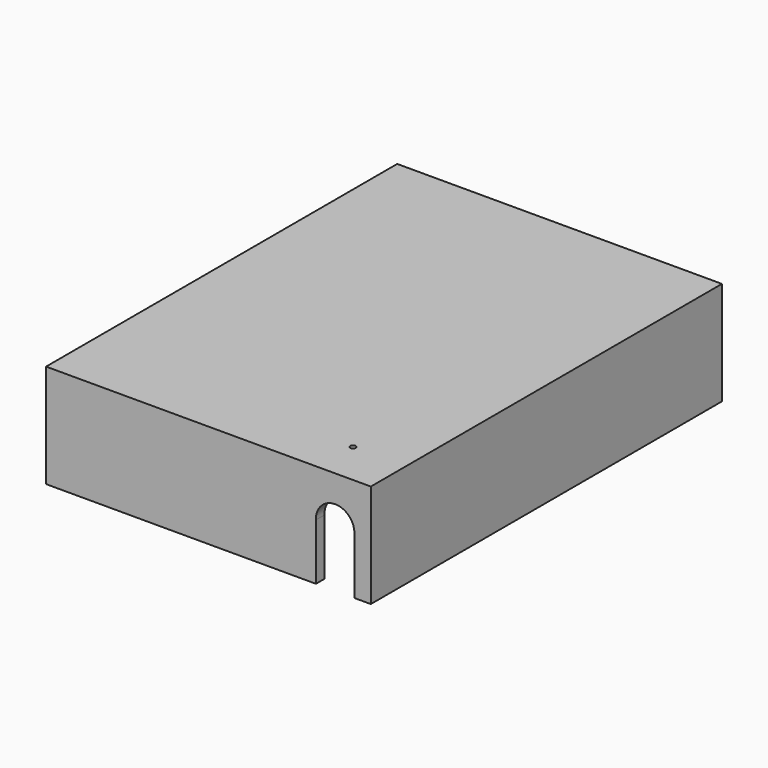
from build123d import *

# Parameters (mm, degrees)
F0_W      = 85
F0_H      = 117
F1_DEPTH  = 4
F2_W      = 2
F2_H      = 5
F3_DEPTH  = 7
F4_W      = 2
F4_H      = 4.0044696238
F5_DEPTH  = 5
F6_R      = 1
F7_R      = 1
F8_R      = 2
F11_W     = 117
F11_H     = 4
F12_DEPTH = 3
F10_W     = 117
F10_H     = 4
F14_DEPTH = 3
F13_W     = 85
F13_H     = 3
F13_W_2   = 3
F13_H_2   = 117
F15_DEPTH = 25
F16_DEPTH = 3
F18_DEPTH = 3
F19_R     = 0.75
F20_DEPTH = 4
F21_DEPTH = 3
F23_DEPTH = 3


# Not quite as in the source:
# - a feature names something its author has since deleted; it is built from what else it names


with BuildPart() as f1:
    # F0 (on Top) → F1 (new body)
    with BuildSketch(Plane.XY):
        Rectangle(F0_W, F0_H)
    extrude(amount=F1_DEPTH)

    # F2 (on face) → F3 (join)
    with BuildSketch(Plane(origin=(0, 0, 0), x_dir=(1, 0, 0), z_dir=(0, 0, -1))):
        with Locations((-21, -36)):
            Rectangle(F2_W, F2_H)
    extrude(amount=F3_DEPTH)

    # F4 (on face) → F5 (join)
    with BuildSketch(Plane(origin=(0, 38.5, 0), x_dir=(-1, 0, 0), z_dir=(0, 1, 0))):
        with Locations((21, -4.9977651881)):
            Rectangle(F4_W, F4_H)
    extrude(amount=F5_DEPTH)

    # F6
    f6_edges = [f1.edges().sort_by_distance(p)[0] for p in [
        (-21, 43.5, -2.99553),
    ]]
    fillet(f6_edges, radius=F6_R)

    # F7
    f7_edges = [f1.edges().sort_by_distance(p)[0] for p in [
        (-21, 43.5, -7),
    ]]
    fillet(f7_edges, radius=F7_R)

    # F8
    f8_edges = [f1.edges().sort_by_distance(p)[0] for p in [
        (-21, 33.5, -7),
    ]]
    fillet(f8_edges, radius=F8_R)


with BuildPart() as f9_1:
    # F9: instance of F1
    add(f1.part.mirror(Plane.YZ))


with BuildPart() as f1_1:
    add(f1.part)

    add(f9_1.part)  # F12 merges F9_1
    # F11 (on face) → F12 (join)
    with BuildSketch(Plane(origin=(-42.5, 0, 0), x_dir=(0, -1, 0), z_dir=(-1, 0, 0))):
        with Locations((0, 2)):
            Rectangle(F11_W, F11_H)
    extrude(amount=F12_DEPTH)

    # F10 (on face) → F14 (join)
    with BuildSketch(Plane.YZ.offset(42.5)):
        with Locations((0, 2)):
            Rectangle(F10_W, F10_H)
    extrude(amount=F14_DEPTH)

    # F13 (on face) → F15 (join)
    with BuildSketch(Plane(origin=(0, 0, 0), x_dir=(1, 0, 0), z_dir=(0, 0, -1))):
        with Locations((0, 60)):
            Rectangle(F13_W, F13_H)
        with Locations((0, -60)):
            Rectangle(F13_W, F13_H)
        with Locations((-44, 0)):
            Rectangle(F13_W_2, F13_H_2)
        with Locations((44, 0)):
            Rectangle(F13_W_2, F13_H_2)
    extrude(amount=F15_DEPTH)

    # F16 (add): a face of the model
    f16_faces = [f1_1.faces().sort_by_distance(p)[0] for p in [
        (0, 58.5, 0.9550916186),
    ]]
    extrude(f16_faces, amount=F16_DEPTH)

    # F17 (on face) → F18 (cut)
    with BuildSketch(Plane(origin=(0, 61.5, 0), x_dir=(-1, 0, 0), z_dir=(0, 1, 0))):
        Polygon((-29.3773965985, -11.6825154486), (-42.3773965985, -11.6825154486), (-42.3773965985, -17.6825154486), (-37.6342944801, -17.6825154486), (-37.6342944801, -20.6825154486), (-34.6342944801, -20.6825154486), (-34.6342944801, -17.6825154486), (-29.3773965985, -17.6825154486), align=None)
    extrude(amount=-F18_DEPTH, mode=Mode.SUBTRACT)

    # F19 (on face) → F20 (cut, through all)
    with BuildSketch(Plane.XY.offset(4)):
        with Locations((30.7380352169, -49.2682121694)):
            Circle(F19_R)
    extrude(amount=-F20_DEPTH, mode=Mode.SUBTRACT)

    # F21 (add): a face of the model
    f21_faces = [f1_1.faces().sort_by_distance(p)[0] for p in [
        (-44.5449083814, -58.5, -10.5),
    ]]
    extrude(f21_faces, amount=F21_DEPTH)

    # F22 (on face) → F23 (cut, through all)
    with BuildSketch(Plane.XZ.offset(61.5)):
        with BuildLine():
            Line((40.9117795325, -25), (40.9117795325, -9.155403553))
            ThreePointArc((40.9117795325, -9.155403553), (35.4678711158, -3.59895141), (30.1197935699, -9.2477004601))
            Line((30.1197935699, -9.2477004601), (30.1197935699, -25))
            Line((30.1197935699, -25), (40.9117795325, -25))
        make_face()
    extrude(amount=-F23_DEPTH, mode=Mode.SUBTRACT)


solid = f1_1.part
